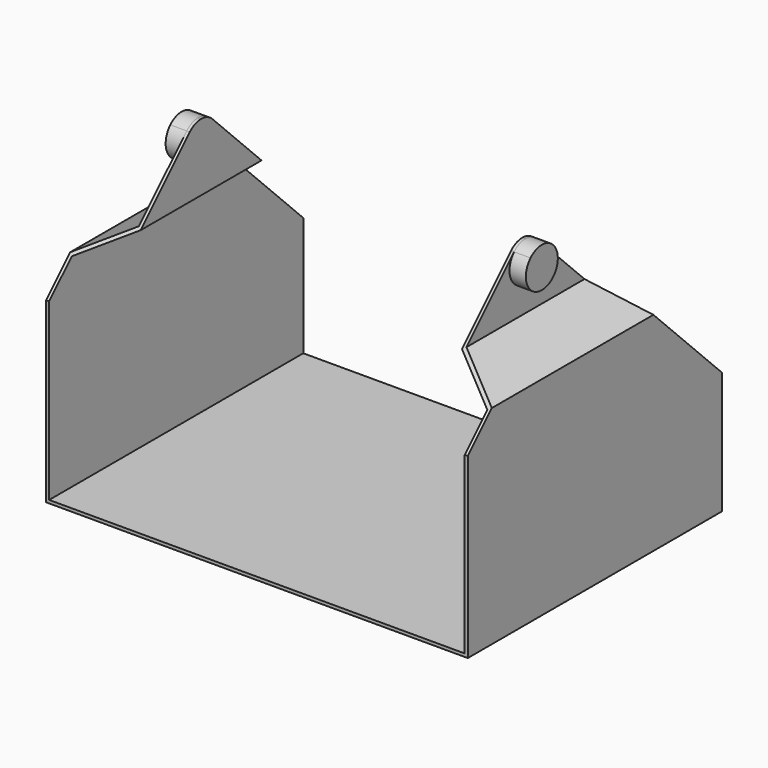
from build123d import *
from build123d import SkipClean  # not in build123d's __all__

# Parameters (mm, degrees)
F1_DEPTH      = 72.39
F1_DEPTH_BACK = 50.8
F2_R          = 7.747
F3_DEPTH      = 69.85
F3_DEPTH_BACK = 69.85
F4_W          = 124.6
F4_H          = 26.092820323
F5_DEPTH      = 72.391
F5_DEPTH_BACK = 50.801
F7_DEPTH      = 81.776
F7_DEPTH_BACK = 81.776


with BuildPart() as f1:
    # F0 (on Front) → F1 (new body, two sides)
    with BuildSketch(Plane.XZ) as f1_sk:
        Polygon((80.575, -36.195), (0, -36.195), (-80.575, -36.195), (-80.575, 42.545), (-62.3, 53.0960761694), (-62.3, 79.1888964925), (-63.5, 79.1888964925), (-63.5, 53.7888964925), (-81.775, 43.237820323), (-81.775, -37.395), (0, -37.395), (81.775, -37.395), (81.775, 43.237820323), (63.5, 53.7888964925), (63.5, 79.1888964925), (62.3, 79.1888964925), (62.3, 53.0960761694), (80.575, 42.545), align=None)
    extrude(amount=-F1_DEPTH)
    extrude(f1_sk.sketch, amount=F1_DEPTH_BACK)

    # F2 (on Right) → F3 (join, two sides)
    with BuildSketch(Plane.YZ) as f3_sk:
        with Locations((0, 71.4418964925)):
            Circle(F2_R)
    extrude(amount=-F3_DEPTH)
    extrude(f3_sk.sketch, amount=F3_DEPTH_BACK)

    # F4 (on Front) → F5 (cut, two sides)
    with BuildSketch(Plane.XZ) as f5_sk:
        with Locations((0, 66.142486331)):
            Rectangle(F4_W, F4_H)
    extrude(amount=-F5_DEPTH, mode=Mode.SUBTRACT)
    extrude(f5_sk.sketch, amount=F5_DEPTH_BACK, mode=Mode.SUBTRACT)

    # F6 (on Right) → F7 (cut, two sides)
    with BuildSketch(Plane.YZ) as f7_sk:
        with BuildLine():
            Line((-50.8, 81.7288964925), (-50.8, 31.5978089602))
            Line((-50.8, 31.5978089602), (-5.4779562339, 76.9198527263))
            ThreePointArc((-5.4779562339, 76.9198527263), (0, 79.1888964925), (5.4779562339, 76.9198527263))
            Line((5.4779562339, 76.9198527263), (72.39, 10.0078089602))
            Line((72.39, 10.0078089602), (72.39, 81.7288964925))
            Line((72.39, 81.7288964925), (-50.8, 81.7288964925))
        make_face()
    with SkipClean():  # cleaning this boolean's faces spoils the solid; the shape is the same uncleaned
        extrude(amount=-F7_DEPTH, mode=Mode.SUBTRACT)
        extrude(f7_sk.sketch, amount=F7_DEPTH_BACK, mode=Mode.SUBTRACT)


solid = f1.part
